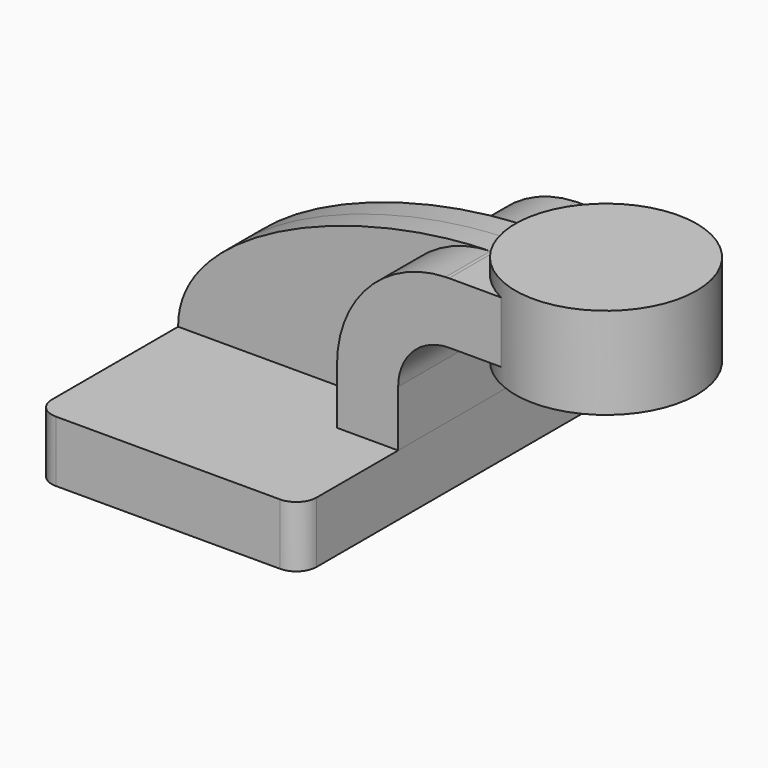
from build123d import *

# Parameters (mm, degrees)
F1_DEPTH = 63.5
F0_W     = 22.5424882722
F0_H     = 19.05
F2_DEPTH = 25.4
F3_DEPTH = 7.9375
F5_R     = 6.35


with BuildPart() as f1:
    # F0 (on Front) → F1 (new body, symmetric)
    with BuildSketch(Plane.XZ):
        Polygon((-41.275, 9.525), (-41.275, -9.525), (41.275, -9.525), (41.275, 9.525), (22.225, 9.525), align=None)
    extrude(amount=F1_DEPTH, both=True)

    # F5
    f5_edges = [f1.edges().sort_by_distance(p)[0] for p in [
        (41.275, -63.5, 0),
        (-41.275, -63.5, 0),
        (41.275, 63.5, 0),
        (-41.275, 63.5, 0),
    ]]
    fillet(f5_edges, radius=F5_R)


with BuildPart() as f2:
    # F0 (on Front) → F2 (new body, symmetric)
    with BuildSketch(Plane.XZ):
        with BuildLine():
            Line((22.225, 9.525), (41.275, 9.525))
            Line((41.275, 9.525), (41.275, 27.0002))
            ThreePointArc((41.275, 27.0002), (45.9246798487, 38.2255201513), (57.15, 42.8752))
            Line((57.15, 42.8752), (63.1825117278, 42.8752))
            Line((63.1825117278, 42.8752), (63.1825117278, 61.9252))
            Line((63.1825117278, 61.9252), (57.15, 61.9252))
            add(Edge.make_bspline(
                [(56.0449542067, 61.9077135006), (56.4140967853, 61.9151121698), (56.7824587666, 61.9209441136), (57.15, 61.9252)],
                knots=[110.563800657, 110.563800657, 110.563800657, 110.563800657, 111.5045361635, 111.5045361635, 111.5045361635, 111.5045361635], degree=3))
            ThreePointArc((56.0449542067, 61.9077135006), (32.0666454663, 51.302071334), (22.225, 27.0002))
            Line((22.225, 27.0002), (22.225, 9.525))
        make_face()
        with Locations((74.4537558639, 52.4002)):
            Rectangle(F0_W, F0_H)
    extrude(amount=F2_DEPTH, both=True)

    # F0 (on Front) → F3 (join, symmetric)
    with BuildSketch(Plane.XZ):
        with BuildLine():
            add(Edge.make_bspline(
                [(-41.275, 9.525), (-41.5074973481, 38.5272765574), (12.65995791, 61.0381545449), (56.0449542067, 61.9077135006)],
                knots=[0, 0, 0, 0, 110.563800657, 110.563800657, 110.563800657, 110.563800657], degree=3))
            Line((-41.275, 9.525), (22.225, 9.525))
            Line((22.225, 9.525), (22.225, 27.0002))
            ThreePointArc((22.225, 27.0002), (32.0666454663, 51.302071334), (56.0449542067, 61.9077135006))
        make_face()
    extrude(amount=F3_DEPTH, both=True)

    # F0 (on Front) → F4 (revolve)
    with BuildSketch(Plane.XZ):
        Polygon((85.725, 66.675), (85.725, 61.9252), (85.725, 42.8752), (85.725, 38.1), (113.9825117278, 38.1), (113.9825117278, 66.675), align=None)
    revolve(axis=Axis((85.725, 0, 52.3875), (0, 0, -1)))


solid = Compound([f1.part, f2.part])
